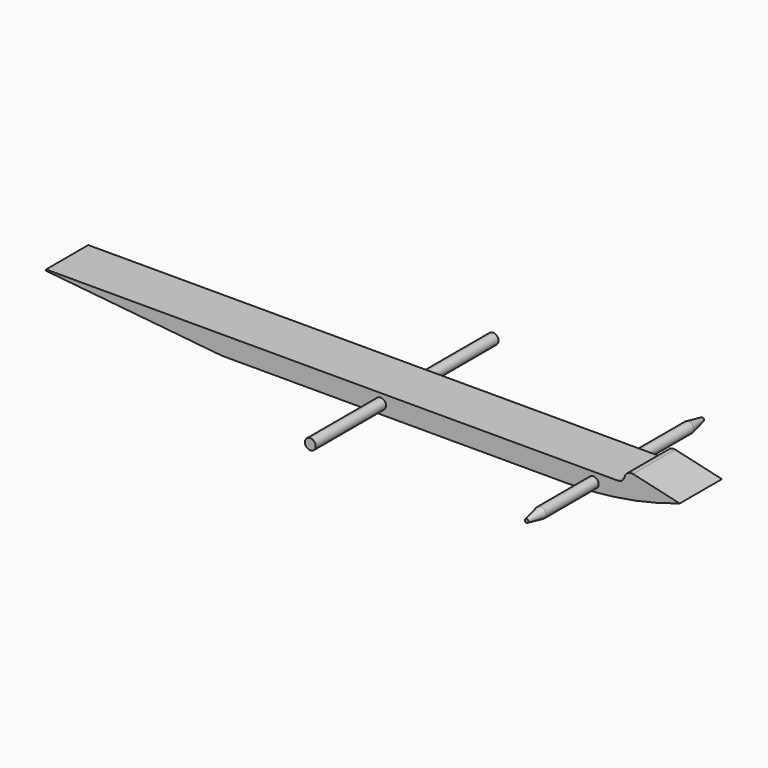
from build123d import *

# Parameters (mm, degrees)
F0_R        = 3.9091582441
F1_DEPTH    = 82.55
F0_R_2      = 3.8256262675
F2_DEPTH    = 79.375
F3_DEPTH    = 19.05
F4_T1_DEPTH = 448.1823504125
F5_R        = 5.08
F6_SIZE2    = 12.7
F6_SIZE     = 127
F7_SIZE2    = 2.54
F7_SIZE     = 12.7


# Not quite as in the source:
# - a fillet or chamfer that OpenCascade refuses, or shapes differently, is made with other operations: its cross-section is extruded or revolved along the edge and cut away or added


with BuildPart() as f1:
    # F0 (on Front) → F1 (new body, symmetric)
    with BuildSketch(Plane.XZ):
        Circle(F0_R)
    extrude(amount=F1_DEPTH, both=True)


with BuildPart() as f2:
    # F0 (on Front) → F2 (new body, symmetric)
    with BuildSketch(Plane.XZ):
        with Locations((153.7049710751, 0)):
            Circle(F0_R_2)
    extrude(amount=F2_DEPTH, both=True)

    # F7
    f7_edges = [f2.edges().sort_by_distance(p)[0] for p in [
        (149.879345, 79.375, 0),
        (149.879345, -79.375, 0),
    ]]
    chamfer(f7_edges, length=F7_SIZE, length2=F7_SIZE2)


with BuildPart() as f3:
    # F0 (on Front) → F3 (new body, symmetric)
    with BuildSketch(Plane.XZ):
        Polygon((-241.6750043631, 6.8029756658), (-241.6750043631, -6.8029756658), (216.0731535405, -6.8029756658), (216.0731535405, 6.8029756658), (175.348284848, 6.8029756658), align=None)
        Circle(F0_R, mode=Mode.SUBTRACT)
        with Locations((153.7049710751, 0)):
            Circle(F0_R_2, mode=Mode.SUBTRACT)
        Polygon((175.348284848, 6.8029756658), (216.0731535405, 6.8029756658), (177.4246394634, 15.7611016184), align=None)
    extrude(amount=F3_DEPTH, both=True)

    # F4: fillet of radius 254 on 1 edges, made by hand

    # F4_s2 → F4_t1 (cut)
    with BuildSketch(Plane.XZ.offset(-224.0911752063)):
        with BuildLine():
            ThreePointArc((216.0731535405, 6.8029756658), (175.6253714227, -3.3784017971), (134.056683458, -6.8029756658))
            Line((134.056683458, -6.8029756658), (216.0731535405, -6.8029756658))
            Line((216.0731535405, -6.8029756658), (216.0731535405, 6.8029756658))
        make_face()
    extrude(amount=F4_T1_DEPTH, mode=Mode.SUBTRACT)

    # F5
    f5_edges = [f3.edges().sort_by_distance(p)[0] for p in [
        (175.348285, 0, 6.802976),
        (177.424639, 0, 15.761102),
    ]]
    fillet(f5_edges, radius=F5_R)

    # F6
    f6_edges = [f3.edges().sort_by_distance(p)[0] for p in [
        (-241.675004, 0, -6.802976),
    ]]
    f6_side = f3.faces().sort_by_distance((-53.80916, 0, -6.802976))[0]
    chamfer(f6_edges, length=F6_SIZE, length2=F6_SIZE2, reference=f6_side)


solid = Compound([f1.part, f2.part, f3.part])
